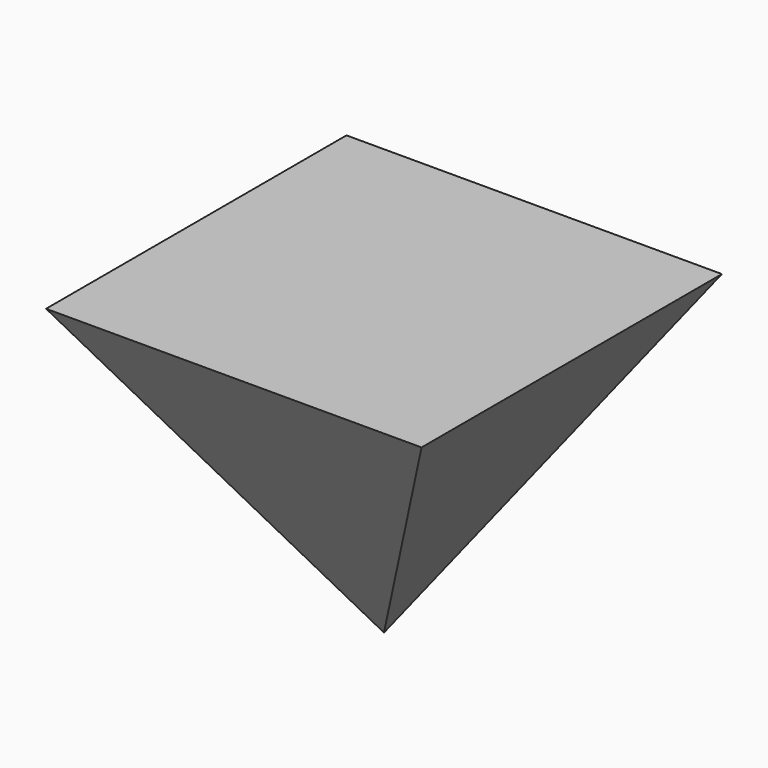
from build123d import *

# Parameters (mm, degrees)
F0_W = 76.2
F0_H = 76.2


# Not quite as in the source:
# - an extrude whose draft closes it to a point is written as a loft to that point


with BuildPart() as f1:
    # F0 (on Top) → F1 section 0
    with BuildSketch(Plane.XY, mode=Mode.PRIVATE) as f1_s0:
        with Locations((27.0737381454, -18.1818129495)):
            Rectangle(F0_W, F0_H)
    loft([f1_s0.sketch, Vertex(27.0737381454, -18.1818129495, -60.9727455565)], ruled=True)


solid = f1.part
